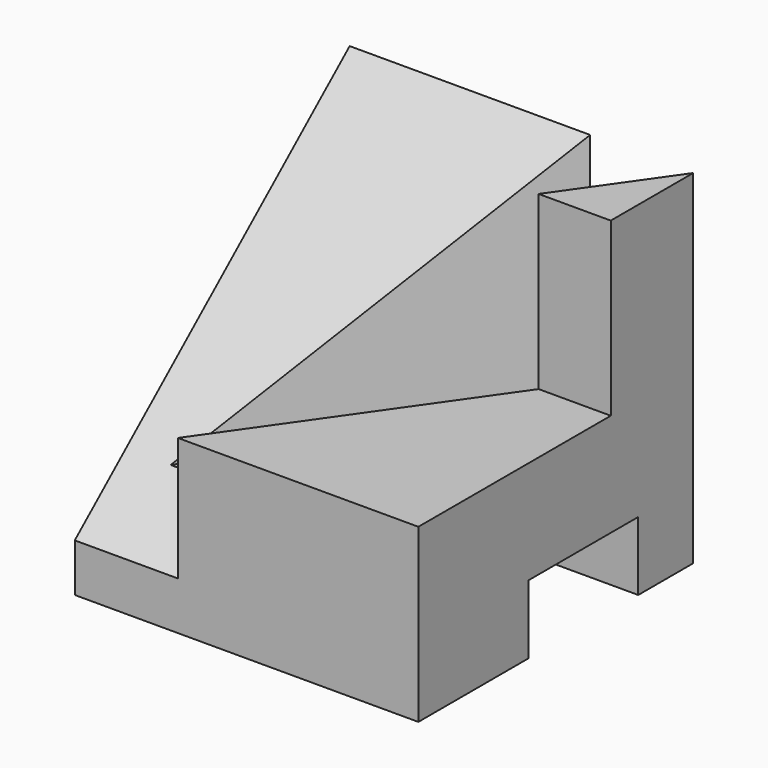
from build123d import *

# Parameters (mm, degrees)
F1_DEPTH  = 50
F4_DEPTH  = 43
F7_REACH  = 115.9479483752
F11_DEPTH = 35
F12_W     = 20
F12_H     = 10
F14_DEPTH = 30


with BuildPart() as f1:
    # F0 (on Right) → F1 (new body)
    with BuildSketch(Plane.YZ):
        Polygon((-50, 0), (0, 0), (0, 50), (-15, 50), (-15, 25), (-50, 25), align=None)
    extrude(amount=-F1_DEPTH)

    # F2 (on face) → F4 (cut, through all)
    with BuildSketch(Plane.XY.offset(50)):
        Polygon((0, 0), (-50, 0), (-50, -50), (-35, -50), align=None)
    extrude(amount=-F4_DEPTH, mode=Mode.SUBTRACT)

    f7_end = Plane(origin=(-13.8970588235, -19.8529411765, 22.3235294118), x_dir=(-0.5734623444, -0.8192319205, 0), z_dir=(-0.8192319205, 0.5734623444, 0))
    # F6 (on plane+point) → F7 (join, up to a plane its end follows)
    with BuildSketch(Plane.YZ.offset(-50)):
        Polygon((-50, 7), (0, 7), (0, 50), align=None)
    f7_long = extrude(amount=F7_REACH, mode=Mode.PRIVATE)
    add(split(f7_long, bisect_by=f7_end, keep=Keep.TOP, mode=Mode.PRIVATE))

    # F9 (on plane+point) → F11 (cut, through all)
    with BuildSketch(Plane.XY.offset(50)):
        Polygon((0, 0), (-15, 0), (-50, -50), (-35, -50), align=None)
    extrude(amount=-F11_DEPTH, mode=Mode.SUBTRACT)

    # F12 (on face) → F14 (cut, through all)
    with BuildSketch(Plane.YZ):
        with Locations((-20, 5)):
            Rectangle(F12_W, F12_H)
    extrude(amount=-F14_DEPTH, mode=Mode.SUBTRACT)


solid = f1.part
